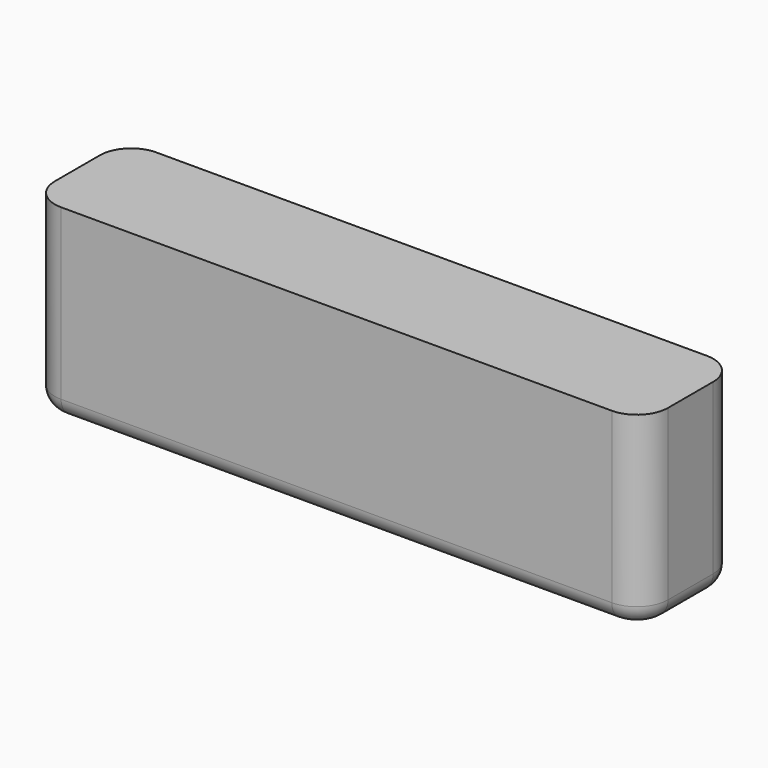
from build123d import *

# Parameters (mm, degrees)
F1_DEPTH = 30
F2_R     = 3


with BuildPart() as f1:
    # F0 (on Top) → F1 (new body)
    with BuildSketch(Plane.XY):
        with BuildLine():
            Line((-44, -9.5), (44, -9.5))
            ThreePointArc((44, -9.5), (47.5355339059, -8.0355339059), (49, -4.5))
            Line((49, -4.5), (49, 4.5))
            ThreePointArc((49, 4.5), (47.5355339059, 8.0355339059), (44, 9.5))
            Line((44, 9.5), (-44, 9.5))
            ThreePointArc((-44, 9.5), (-47.5355339059, 8.0355339059), (-49, 4.5))
            Line((-49, 4.5), (-49, -4.5))
            ThreePointArc((-49, -4.5), (-47.5355339059, -8.0355339059), (-44, -9.5))
        make_face()
    extrude(amount=F1_DEPTH)

    # F2
    f2_edges = [f1.edges().sort_by_distance(p)[0] for p in [
        (0, -9.5, 0),
        (47.535534, -8.035534, 0),
        (49, 0, 0),
        (47.535534, 8.035534, 0),
        (0, 9.5, 0),
        (-47.535534, 8.035534, 0),
        (-49, 0, 0),
        (-47.535534, -8.035534, 0),
    ]]
    fillet(f2_edges, radius=F2_R)


solid = f1.part
